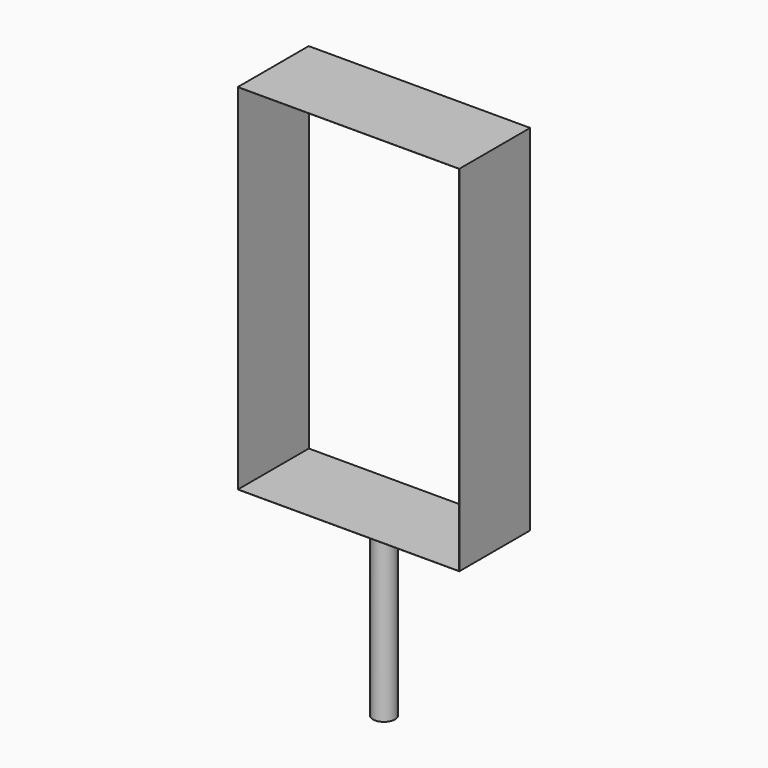
from build123d import *

# Parameters (mm, degrees)
F0_R     = 76.2
F1_DEPTH = 1219.2
F3_W     = 1524
F3_H     = 609.6
F4_DEPTH = 2438.4
F5_T     = -1


# Not quite as in the source:
# - the program builds the solid bodies; features that only make, move or delete a surface that nothing else refers to are left out


with BuildPart() as f1:
    # F0 (on Top) → F1 (new body)
    with BuildSketch(Plane.XY):
        Circle(F0_R)
    extrude(amount=F1_DEPTH)


with BuildPart() as f4:
    # F3 (on offset) → F4 (new body)
    with BuildSketch(Plane.XY.offset(1244.2)):
        Rectangle(F3_W, F3_H)
    extrude(amount=F4_DEPTH)

    # F5
    f5_openings = [f4.faces().sort_by_distance(p)[0] for p in [
        (0, -304.8, 2463.4),
        (0, 304.8, 2463.4),
    ]]
    offset(amount=F5_T, openings=f5_openings)


solid = Compound([f1.part, f4.part])
